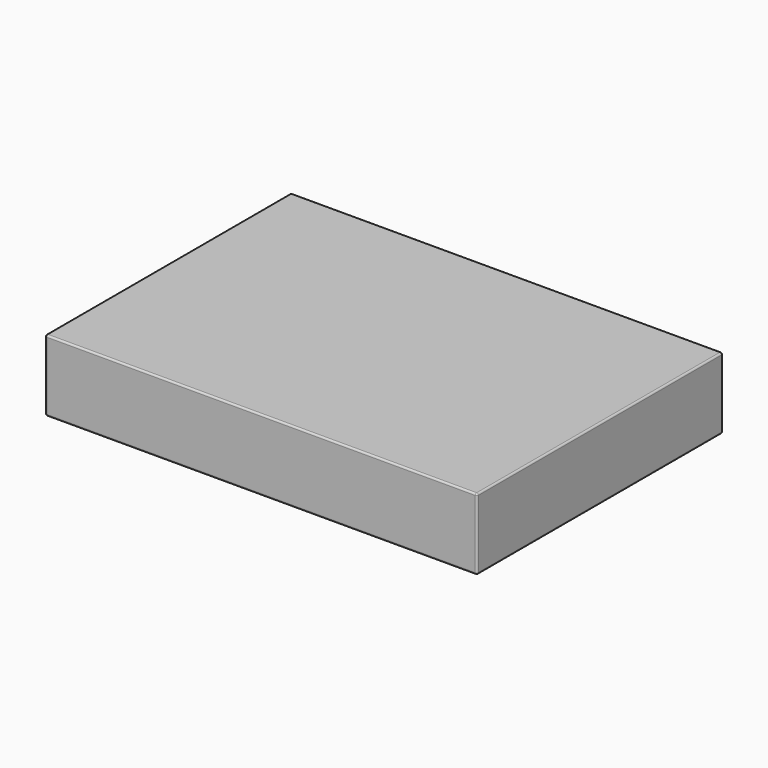
from build123d import *

# Parameters (mm, degrees)
F0_W     = 248
F0_H     = 176.5
F1_DEPTH = 41
F3_T     = -2.5
F4_R     = 1


with BuildPart() as f1:
    # F0 (on Top) → F1 (new body)
    with BuildSketch(Plane.XY):
        with Locations((124, 88.25)):
            Rectangle(F0_W, F0_H)
    extrude(amount=F1_DEPTH)

    # F3
    f3_openings = [f1.faces().sort_by_distance(p)[0] for p in [
        (0, 88.25, 20.5),
    ]]
    offset(amount=F3_T, openings=f3_openings)

    # F4
    f4_edges = [f1.edges().sort_by_distance(p)[0] for p in [
        (124, 176.5, 41),
        (124, 176.5, 0),
        (0, 176.5, 20.5),
        (0, 88.25, 0),
        (0, 88.25, 41),
        (124, 0, 41),
        (0, 0, 20.5),
        (124, 0, 0),
        (248, 0, 20.5),
        (248, 88.25, 41),
        (248, 88.25, 0),
        (248, 176.5, 20.5),
    ]]
    fillet(f4_edges, radius=F4_R)


solid = f1.part
